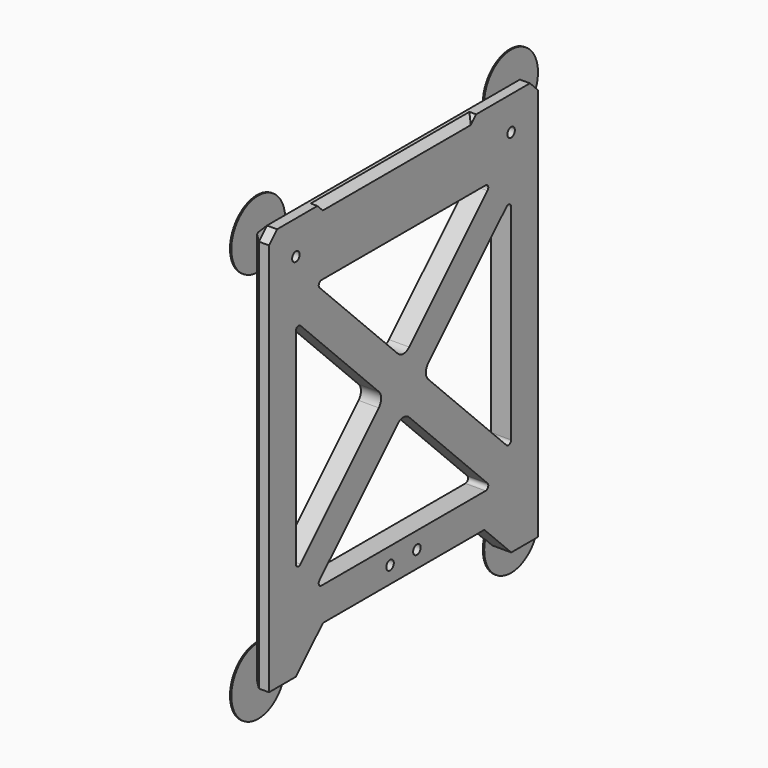
from build123d import *

# Parameters (mm, degrees)
F1_DEPTH       = 6
F2_R           = 1
F3_D           = 2.8
F3_CBORE_D     = 6
F3_CBORE_DEPTH = 2.5
F4_R           = 5
F5_DEPTH       = 1.8
F7_D           = 2.8
F7_CBORE_D     = 6
F7_CBORE_DEPTH = 2.5
F8_SIZE        = 3
F10_DEPTH      = 0.4
F11_W          = 2
F11_H          = 59
F12_DEPTH      = 2
F13_SIZE       = 1.99999


# Not quite as in the source:
# - a fillet or chamfer is up to 0.001 mm smaller than in the source, because OpenCascade refuses the exact size


with BuildPart() as f1:
    # F0 (on Right) → F1 (new body)
    with BuildSketch(Plane.YZ):
        Polygon((40.0512183458, -60), (50, -60), (50, 60), (-50, 60), (-50, -60), (-40, -60), (-29.9487816542, -50), (30.0512183458, -50), align=None)
        with BuildLine():
            Line((2.1213203436, -9.1923881554), (32.9289321881, -40))
            Line((32.9289321881, -40), (-32.9289321881, -40))
            Line((-32.9289321881, -40), (-2.1213203436, -9.1923881554))
            ThreePointArc((-2.1213203436, -9.1923881554), (0, -8.313708499), (2.1213203436, -9.1923881554))
        make_face(mode=Mode.SUBTRACT)
        with BuildLine():
            Line((-9.1923881554, -2.1213203436), (-40, -32.9289321881))
            Line((-40, -32.9289321881), (-40, 32.9289321881))
            Line((-40, 32.9289321881), (-9.1923881554, 2.1213203436))
            ThreePointArc((-9.1923881554, 2.1213203436), (-8.313708499, 0), (-9.1923881554, -2.1213203436))
        make_face(mode=Mode.SUBTRACT)
        with BuildLine():
            Line((40, 32.9289321881), (40, -32.9289321881))
            Line((40, -32.9289321881), (9.1923881554, -2.1213203436))
            ThreePointArc((9.1923881554, -2.1213203436), (8.313708499, 0), (9.1923881554, 2.1213203436))
            Line((9.1923881554, 2.1213203436), (40, 32.9289321881))
        make_face(mode=Mode.SUBTRACT)
        with BuildLine():
            Line((-32.9289321881, 40), (32.9289321881, 40))
            Line((32.9289321881, 40), (2.1213203436, 9.1923881554))
            ThreePointArc((2.1213203436, 9.1923881554), (0, 8.313708499), (-2.1213203436, 9.1923881554))
            Line((-2.1213203436, 9.1923881554), (-32.9289321881, 40))
        make_face(mode=Mode.SUBTRACT)
    extrude(amount=F1_DEPTH)

    # F2
    f2_edges = [f1.edges().sort_by_distance(p)[0] for p in [
        (3, -32.928932, 40),
        (3, 32.928932, 40),
        (3, -40, 32.928932),
        (3, -40, -32.928932),
        (3, -32.928932, -40),
        (3, 40, 32.928932),
        (3, 40, -32.928932),
        (3, 32.928932, -40),
    ]]
    fillet(f2_edges, radius=F2_R)

    # F3 (through all)
    with Locations(Plane(origin=(0, 0, 0), x_dir=(0, 1, 0), z_dir=(-1, 0, 0))):
        with Locations((-40, -50), (40, -50)):
            CounterBoreHole(F3_D / 2, F3_CBORE_D / 2, F3_CBORE_DEPTH)

    # F4 (on face) → F5 (cut)
    with BuildSketch(Plane(origin=(0, 0, 0), x_dir=(0, -1, 0), z_dir=(-1, 0, 0))):
        Circle(F4_R)
    extrude(amount=-F5_DEPTH, mode=Mode.SUBTRACT)

    # F7 (through all)
    with Locations(Plane(origin=(0, 0, 0), x_dir=(0, -1, 0), z_dir=(-1, 0, 0))):
        with Locations((-5, -45), (5, -45)):
            CounterBoreHole(F7_D / 2, F7_CBORE_D / 2, F7_CBORE_DEPTH)

    # F8
    f8_edges = [f1.edges().sort_by_distance(p)[0] for p in [
        (3, -50, 60),
        (3, 50, 60),
        (0, -50, 0),
        (0, 50, 0),
        (0, 0, 60),
    ]]
    chamfer(f8_edges, length=F8_SIZE)

    # F9 (on face) → F10 (join)
    with BuildSketch(Plane(origin=(0, 0, 0), x_dir=(0, -1, 0), z_dir=(-1, 0, 0))):
        with BuildLine():
            Line((-47, 57), (-37, 57))
            ThreePointArc((-37, 57), (-54.0710678119, 64.0710678119), (-47, 47))
            Line((-47, 47), (-47, 57))
        make_face()
        with BuildLine():
            ThreePointArc((47, 47), (54.0710678119, 64.0710678119), (37, 57))
            Line((37, 57), (47, 57))
            Line((47, 57), (47, 47))
        make_face()
        with BuildLine():
            Line((-47, -60), (-47, -50))
            ThreePointArc((-47, -50), (-53.0480452096, -67.9637396456), (-37.3669885172, -57.3157701715))
            Line((-37.3669885172, -57.3157701715), (-40.0512183458, -60))
            Line((-40.0512183458, -60), (-47, -60))
        make_face()
        with BuildLine():
            ThreePointArc((37.3529996858, -57.3664880981), (53.0689735945, -67.9478021811), (47, -50))
            Line((47, -50), (47, -60))
            Line((47, -60), (40, -60))
            Line((40, -60), (37.3529996858, -57.3664880981))
        make_face()
    extrude(amount=-F10_DEPTH)

    # F11 (on face) → F12 (cut)
    with BuildSketch(Plane.XY.offset(60)):
        with Locations((5, -2.5)):
            Rectangle(F11_W, F11_H)
    extrude(amount=-F12_DEPTH, mode=Mode.SUBTRACT)

    # F13 (size 2 in the source; OpenCascade refuses exactly that, so slightly less here)
    f13_edges = [f1.edges().sort_by_distance(p)[0] for p in [
        (4, -2.5, 58),
        (5, 27, 58),
        (5, -32, 58),
    ]]
    chamfer(f13_edges, length=F13_SIZE)


solid = f1.part
